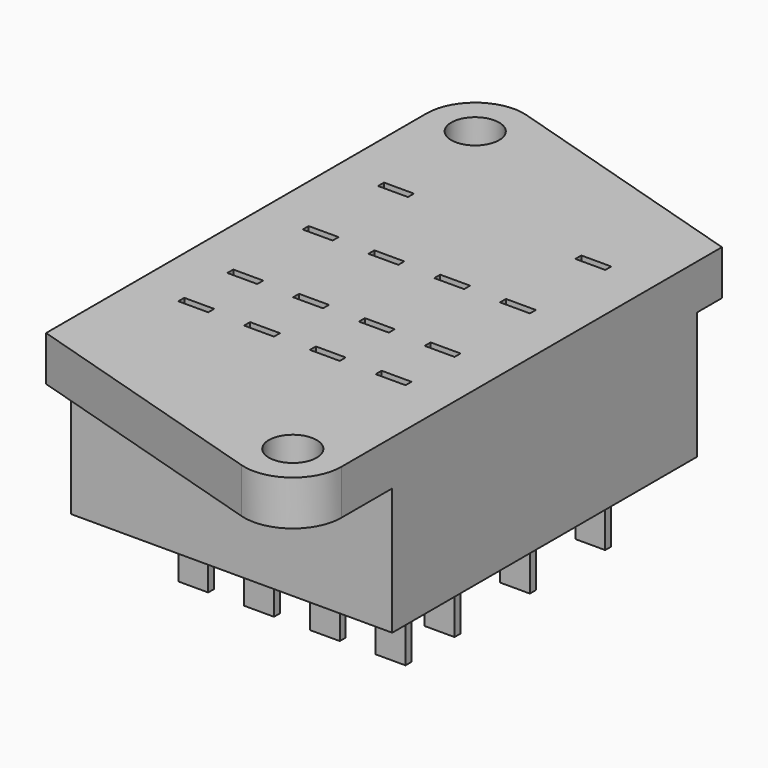
from build123d import *

# Parameters (mm, degrees)
F0_R     = 1.6
F1_DEPTH = 3
F2_W     = 21.5
F2_H     = 25.5
F3_DEPTH = 8.5
F4_W     = 2
F4_H     = 0.5
F5_DEPTH = 5
F6_START = -6
F6_DEPTH = 5.5
F7_R     = 2.3749
F7_R_2   = 1.27
F8_DEPTH = 19.05


with BuildPart() as f1:
    # F0 (on Top) → F1 (new body)
    with BuildSketch(Plane.XY):
        with BuildLine():
            ThreePointArc((-6.5497919597, 20.1079904569), (-9.4331740569, 19.612534797), (-10.75, 17))
            Line((-10.75, 17), (-10.75, -14.818913272))
            Line((-10.75, -14.818913272), (6.5497919597, -20.1079904569))
            ThreePointArc((6.5497919597, -20.1079904569), (9.4331740569, -19.612534797), (10.75, -17))
            Line((10.75, -17), (10.75, 14.818913272))
            Line((10.75, 14.818913272), (-6.5497919597, 20.1079904569))
        make_face()
        with Locations((7.5, -17)):
            Circle(F0_R, mode=Mode.SUBTRACT)
        with Locations((-7.5, 17)):
            Circle(F0_R, mode=Mode.SUBTRACT)
    extrude(amount=F1_DEPTH)

    # F2 (on Top) → F3 (join)
    with BuildSketch(Plane.XY):
        Rectangle(F2_W, F2_H)
    extrude(amount=-F3_DEPTH)

    # F4 (on face) → F5 (join)
    with BuildSketch(Plane(origin=(0, 0, -8.5), x_dir=(1, 0, 0), z_dir=(0, 0, -1))):
        with Locations((-6.6, 7.45)):
            Rectangle(F4_W, F4_H)
        with Locations((-2.2, 7.45)):
            Rectangle(F4_W, F4_H)
        with Locations((2.2, 7.45)):
            Rectangle(F4_W, F4_H)
        with Locations((6.6, 7.45)):
            Rectangle(F4_W, F4_H)
        with Locations((6.6, 3.35)):
            Rectangle(F4_W, F4_H)
        with Locations((-6.6, 3.35)):
            Rectangle(F4_W, F4_H)
        with Locations((-2.2, 3.35)):
            Rectangle(F4_W, F4_H)
        with Locations((2.2, 3.35)):
            Rectangle(F4_W, F4_H)
        with Locations((2.2, -2.95)):
            Rectangle(F4_W, F4_H)
        with Locations((-2.2, -2.95)):
            Rectangle(F4_W, F4_H)
        with Locations((6.6, -2.95)):
            Rectangle(F4_W, F4_H)
        with Locations((-6.6, -2.95)):
            Rectangle(F4_W, F4_H)
        with Locations((6.6, -9.25)):
            Rectangle(F4_W, F4_H)
        with Locations((-6.6, -9.25)):
            Rectangle(F4_W, F4_H)
    extrude(amount=F5_DEPTH)

    # F4 (on face) → F6 (cut)
    with BuildSketch(Plane(origin=(0, 0, -8.5), x_dir=(1, 0, 0), z_dir=(0, 0, -1)).offset(F6_START)):
        with Locations((-6.6, 7.45)):
            Rectangle(F4_W, F4_H)
        with Locations((-2.2, 7.45)):
            Rectangle(F4_W, F4_H)
        with Locations((2.2, 7.45)):
            Rectangle(F4_W, F4_H)
        with Locations((6.6, 7.45)):
            Rectangle(F4_W, F4_H)
        with Locations((6.6, 3.35)):
            Rectangle(F4_W, F4_H)
        with Locations((-6.6, 3.35)):
            Rectangle(F4_W, F4_H)
        with Locations((-2.2, 3.35)):
            Rectangle(F4_W, F4_H)
        with Locations((2.2, 3.35)):
            Rectangle(F4_W, F4_H)
        with Locations((2.2, -2.95)):
            Rectangle(F4_W, F4_H)
        with Locations((-2.2, -2.95)):
            Rectangle(F4_W, F4_H)
        with Locations((6.6, -2.95)):
            Rectangle(F4_W, F4_H)
        with Locations((-6.6, -2.95)):
            Rectangle(F4_W, F4_H)
        with Locations((6.6, -9.25)):
            Rectangle(F4_W, F4_H)
        with Locations((-6.6, -9.25)):
            Rectangle(F4_W, F4_H)
    extrude(amount=-F6_DEPTH, mode=Mode.SUBTRACT)


with BuildPart() as f8:
    # F7 (on Top) → F8 (new body)
    with BuildSketch(Plane.XY):
        with Locations((-7.5, 17)):
            Circle(F7_R)
        with Locations((-7.5, 17)):
            Circle(F7_R_2, mode=Mode.SUBTRACT)
    extrude(amount=-F8_DEPTH)


solid = Compound([f1.part, f8.part])
